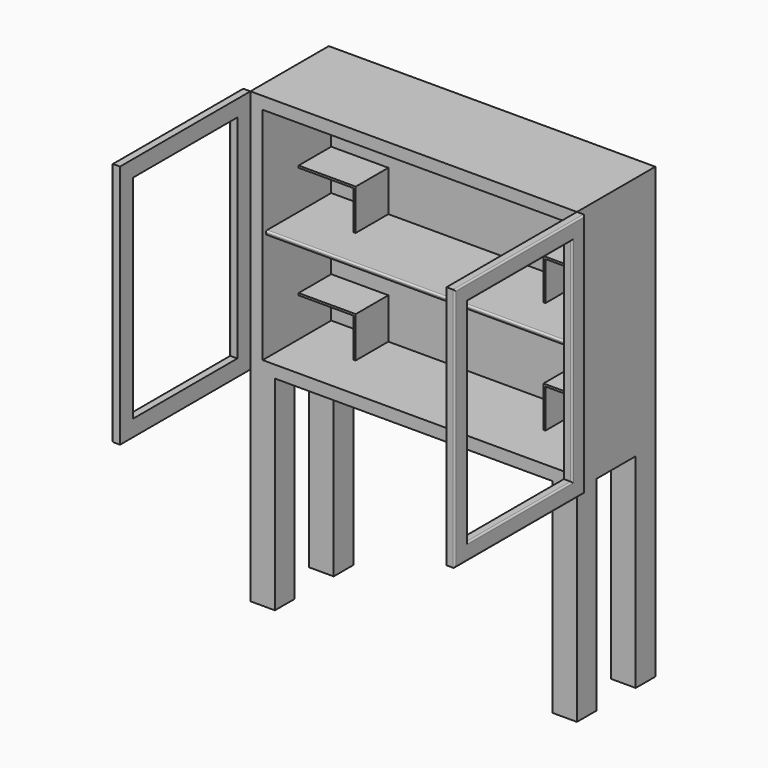
from build123d import *

# Parameters (mm, degrees)
F0_W               = 1016
F0_H               = 304.8
F1_DEPTH           = 762
F2_W               = 76.2
F2_H               = 76.2
F3_DEPTH           = 635
F4_T               = 38.1
F4_T3_DEPTH        = 152.4
F4_T5_DEPTH        = 152.4
F4_T7_DEPTH        = 152.4
F4_T9_DEPTH        = 152.4
F6_E14_W           = 939.8
F6_E14_H           = 254
F7_DEPTH           = 6.35
F10_E15_W          = 177.8
F10_E15_H          = 127
F10_E19_W          = 177.8
F10_E19_H          = 127
F10_E17_MIRRORCS_W = 177.8
F10_E17_MIRRORCS_H = 127
F10_E21_MIRRORCS_W = 177.8
F10_E21_MIRRORCS_H = 127
F11_DEPTH          = 6.35
F10_E16_W          = 127
F10_E16_H          = 127
F10_E20_W          = 127
F10_E20_H          = 127
F12_DEPTH          = 6.35
F10_E18_MIRRORCS_W = 127
F10_E18_MIRRORCS_H = 127
F10_E22_MIRRORCS_W = 127
F10_E22_MIRRORCS_H = 127
F13_DEPTH          = 6.35
F15_W              = 507.20625
F15_H              = 762
F16_DEPTH          = 25.4
F17_W              = 405.60625
F17_H              = 660.4
F18_DEPTH          = 25.4
F19_R              = 5.08
F21_R              = 5.08


# Not quite as in the source:
# - a shell that OpenCascade refuses in one call is made with other operations: the cavity is built on its own and cut out


with BuildPart() as f1:
    # F0 (on Top) → F1 (new body)
    with BuildSketch(Plane.XY):
        Rectangle(F0_W, F0_H)
    extrude(amount=F1_DEPTH)

    # F2 (on face) → F3 (join)
    with BuildSketch(Plane(origin=(0, 0, 0), x_dir=(1, 0, 0), z_dir=(0, 0, -1))):
        with Locations((469.9, 114.3)):
            Rectangle(F2_W, F2_H)
        with Locations((469.9, -114.3)):
            Rectangle(F2_W, F2_H)
        with Locations((-469.9, 114.3)):
            Rectangle(F2_W, F2_H)
        with Locations((-469.9, -114.3)):
            Rectangle(F2_W, F2_H)
    extrude(amount=F3_DEPTH)

    # F4: shell of thickness 38.1, made by hand


with BuildPart() as f4_core1:
    # F4_t2: copy of F1
    add(f1.part)

    # the walls: a layer under each face that stays
    f4_faces = [f4_core1.faces().sort_by_distance(p)[0] for p in [
        (-469.9, -114.3, -635),
        (-469.9, -76.2, -317.5),
        (-431.8, -114.3, -317.5),
        (0, 0, 0),
        (469.9, -76.2, -317.5),
        (469.9, 76.2, -317.5),
        (469.9, 114.3, -635),
        (431.8, 114.3, -317.5),
        (0, 152.4, 63.5),
        (-469.9, 114.3, -635),
        (-431.8, 114.3, -317.5),
        (-469.9, 76.2, -317.5),
        (431.8, -114.3, -317.5),
        (469.9, -114.3, -635),
        (508, 0, 63.5),
        (0, 0, 762),
        (-508, 0, 63.5),
    ]]
    thicken(f4_faces, amount=-F4_T, mode=Mode.SUBTRACT)

    # F4_s4 → F4_t3 (cut)
    with BuildSketch(Plane.YZ.offset(-546.1)):
        Polygon((-75.819, -0.381), (-114.3, 0), (-114.3, 38.1), (-76.2, 38.1), align=None)
        Polygon((75.819, -0.381), (76.2, 38.1), (114.3, 38.1), (114.3, 0), align=None)
    extrude(amount=F4_T3_DEPTH, mode=Mode.SUBTRACT)

    # F4_s6 → F4_t5 (cut)
    with BuildSketch(Plane.XZ.offset(38.1)):
        Polygon((-431.419, -0.381), (-469.9, 0), (-469.9, 38.1), (-431.8, 38.1), align=None)
        Polygon((431.419, -0.381), (431.8, 38.1), (469.9, 38.1), (469.9, 0), align=None)
    extrude(amount=F4_T5_DEPTH, mode=Mode.SUBTRACT)

    # F4_s8 → F4_t7 (cut)
    with BuildSketch(Plane.XZ.offset(-190.5)):
        Polygon((-431.419, -0.381), (-431.8, 38.1), (-469.9, 38.1), (-469.9, 0), align=None)
        Polygon((431.419, -0.381), (431.8, 38.1), (469.9, 38.1), (469.9, 0), align=None)
    extrude(amount=F4_T7_DEPTH, mode=Mode.SUBTRACT)

    # F4_s10 → F4_t9 (cut)
    with BuildSketch(Plane.YZ.offset(393.7)):
        Polygon((75.819, -0.381), (76.2, 38.1), (114.3, 38.1), (114.3, 0), align=None)
        Polygon((-75.819, -0.381), (-76.2, 38.1), (-114.3, 38.1), (-114.3, 0), align=None)
    extrude(amount=F4_T9_DEPTH, mode=Mode.SUBTRACT)


with BuildPart() as f1_1:
    add(f1.part)

    # what is left inside the walls is the cavity
    f4_cavity = [f4_core1.part.solids().sort_by_distance(p)[0] for p in [
        (0, -152.019, 495.3),
    ]]
    add(f4_cavity, mode=Mode.SUBTRACT)

    # F6_E14 (on explicit) → F7 (join, symmetric)
    with BuildSketch(Plane(origin=(-469.9, 114.3, 381), x_dir=(1, 0, 0), z_dir=(0, 0, -1))):
        with Locations((469.9, 127)):
            Rectangle(F6_E14_W, F6_E14_H)
    extrude(amount=F7_DEPTH, both=True)

    # F10_E15 (on explicit) + F10_E19 (on explicit) + F10_E17_MirrorCS (on explicit) + F10_E21_MirrorCS (on explicit) → F11 (join)
    with BuildSketch(Plane(origin=(-469.9, 114.3, 514.35), x_dir=(1, 0, 0), z_dir=(0, 0, -1))):
        with Locations((88.9, 63.5)):
            Rectangle(F10_E15_W, F10_E15_H)
    with BuildSketch(Plane(origin=(-469.9, 114.3, 165.1), x_dir=(1, 0, 0), z_dir=(0, 0, -1))):
        with Locations((88.9, 63.5)):
            Rectangle(F10_E19_W, F10_E19_H)
    with BuildSketch(Plane(origin=(469.9, 114.3, 514.35), x_dir=(-1, 0, 0), z_dir=(0, 0, 1))):
        with Locations((88.9, 63.5)):
            Rectangle(F10_E17_MIRRORCS_W, F10_E17_MIRRORCS_H)
    with BuildSketch(Plane(origin=(469.9, 114.3, 165.1), x_dir=(-1, 0, 0), z_dir=(0, 0, 1))):
        with Locations((88.9, 63.5)):
            Rectangle(F10_E21_MIRRORCS_W, F10_E21_MIRRORCS_H)
    extrude(amount=F11_DEPTH, dir=(0, 0, -1))

    # F10_E16 (on explicit) + F10_E20 (on explicit) → F12 (join)
    with BuildSketch(Plane(origin=(-292.1, 114.3, 514.35), x_dir=(0, 0, -1), z_dir=(-1, 0, 0))):
        with Locations((63.5, 63.5)):
            Rectangle(F10_E16_W, F10_E16_H)
    with BuildSketch(Plane(origin=(-292.1, 114.3, 165.1), x_dir=(0, 0, -1), z_dir=(-1, 0, 0))):
        with Locations((63.5, 63.5)):
            Rectangle(F10_E20_W, F10_E20_H)
    extrude(amount=F12_DEPTH)

    # F10_E18_MirrorCS (on explicit) + F10_E22_MirrorCS (on explicit) → F13 (join)
    with BuildSketch(Plane(origin=(292.1, 114.3, 514.35), x_dir=(0, 0, -1), z_dir=(-1, 0, 0))):
        with Locations((63.5, 63.5)):
            Rectangle(F10_E18_MIRRORCS_W, F10_E18_MIRRORCS_H)
    with BuildSketch(Plane(origin=(292.1, 114.3, 165.1), x_dir=(0, 0, -1), z_dir=(-1, 0, 0))):
        with Locations((63.5, 63.5)):
            Rectangle(F10_E22_MIRRORCS_W, F10_E22_MIRRORCS_H)
    extrude(amount=-F13_DEPTH)

    # F21
    f21_edges = [f1_1.edges().sort_by_distance(p)[0] for p in [
        (0, -139.7, 374.65),
        (0, -139.7, 387.35),
    ]]
    fillet(f21_edges, radius=F21_R)


with BuildPart() as f16:
    # F15 (on offset) → F16 (new body)
    with BuildSketch(Plane.YZ.offset(508)):
        with Locations((-406.003125, 381)):
            Rectangle(F15_W, F15_H)
    extrude(amount=F16_DEPTH)

    # F17 (on face) → F18 (cut)
    with BuildSketch(Plane.YZ.offset(533.4)):
        with Locations((-406.003125, 381)):
            Rectangle(F17_W, F17_H)
    extrude(amount=-F18_DEPTH, mode=Mode.SUBTRACT)

    # F19
    f19_edges = [f16.edges().sort_by_distance(p)[0] for p in [
        (533.4, -152.4, 381),
        (533.4, -406.003125, 0),
        (533.4, -406.003125, 762),
        (533.4, -659.60625, 381),
        (533.4, -406.003125, 50.8),
        (533.4, -203.2, 381),
        (533.4, -406.003125, 711.2),
        (533.4, -608.80625, 381),
    ]]
    fillet(f19_edges, radius=F19_R)


with BuildPart() as f20_1:
    # F20: instance of F16
    add(f16.part.mirror(Plane.YZ))


solid = Compound([f1_1.part, f16.part, f20_1.part])
